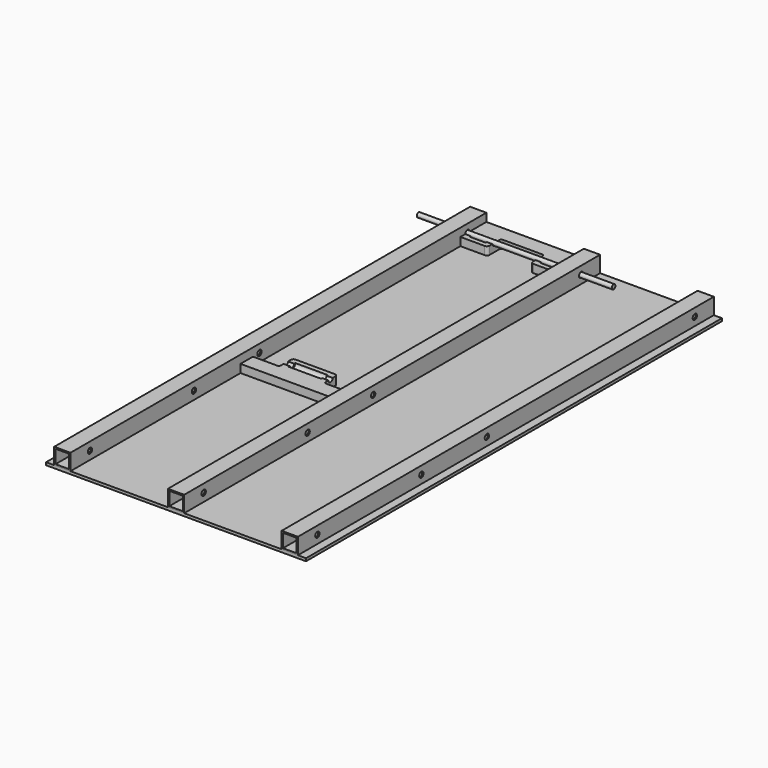
from build123d import *

# Parameters (mm, degrees)
F0_W      = 1219.2
F0_H      = 2438.4
F1_DEPTH  = 12.7
F2_W      = 76.2
F2_H      = 76.2
F2_W_2    = 63.5
F2_H_2    = 63.5
F3_DEPTH  = 1219.2
F5_DEPTH  = 76.2
F6_R      = 12.7
F7_DEPTH  = 609.6
F8_R      = 9.525
F8_2_R    = 9.525
F9_R      = 12.7
F9_2_R    = 12.7
F11_R     = 10.668
F12_DEPTH = 457.2
F14_W     = 1451.5540599823
F14_H     = 2822.6795196533
F15_DEPTH = 38.101
F17_R     = 19.05
F18_DEPTH = 38.1
F19_R     = 3.175
F20_R     = 19.05
F21_DEPTH = 76.2


# Not quite as in the source:
# - a pattern or mirror of a feature is missing from the dataset's text; its kind, count and spacing are read off the source's solid


with BuildPart() as f1:
    # F0 (on Top) → F1 (new body)
    with BuildSketch(Plane.XY):
        Rectangle(F0_W, F0_H)
    extrude(amount=F1_DEPTH)


with BuildPart() as f3:
    # F2 (on Front) → F3 (new body, symmetric)
    with BuildSketch(Plane.XZ):
        with Locations((0, 50.8)):
            Rectangle(F2_W, F2_H)
        with Locations((0, 50.8)):
            Rectangle(F2_W_2, F2_H_2, mode=Mode.SUBTRACT)
    extrude(amount=F3_DEPTH, both=True)


with BuildPart() as f3b:
    # F2 (on Front) → F3, piece 2 (new body, symmetric)
    with BuildSketch(Plane.XZ):
        with Locations((-533.4, 50.8)):
            Rectangle(F2_W, F2_H)
        with Locations((-533.4, 50.8)):
            Rectangle(F2_W_2, F2_H_2, mode=Mode.SUBTRACT)
    extrude(amount=F3_DEPTH, both=True)


with BuildPart() as f3c:
    # F2 (on Front) → F3, piece 3 (new body, symmetric)
    with BuildSketch(Plane.XZ):
        with Locations((533.4, 50.8)):
            Rectangle(F2_W, F2_H)
        with Locations((533.4, 50.8)):
            Rectangle(F2_W_2, F2_H_2, mode=Mode.SUBTRACT)
    extrude(amount=F3_DEPTH, both=True)


with BuildPart() as f5:
    # F4 (on face) → F5 (new body, through all)
    with BuildSketch(Plane.XY.offset(12.7)):
        Polygon((-495.3, 1219.2), (-495.3, 1066.8), (-368.3, 1066.8), (-368.3, 1146.175), (-165.1, 1146.175), (-165.1, 1066.8), (-38.1, 1066.8), (-38.1, 1219.2), align=None)
    extrude(amount=F5_DEPTH)


with BuildPart() as f5b:
    # F4 (on face) → F5, piece 2 (new body, through all)
    with BuildSketch(Plane.XY.offset(12.7)):
        Polygon((-495.3, -149.225), (-495.3, -222.25), (-38.1, -222.25), (-38.1, -149.225), (-161.925, -149.225), (-161.925, -69.85), (-371.475, -69.85), (-371.475, -149.225), align=None)
    extrude(amount=F5_DEPTH)


with BuildPart() as f7_tool:
    # F6 (on Right) → F7 (new body, symmetric)
    with BuildSketch(Plane.YZ):
        with Locations((1108.075, 50.8)):
            Circle(F6_R)
        with Locations((-111.125, 50.8)):
            Circle(F6_R)
        with Locations((-495.3, 50.8)):
            Circle(F6_R)
        with Locations((-1104.9, 50.8)):
            Circle(F6_R)
    extrude(amount=F7_DEPTH, both=True)


with BuildPart() as f3_1:
    add(f3.part)

    # F7: cut by f7_tool
    add(f7_tool.part, mode=Mode.SUBTRACT)


with BuildPart() as f3b_1:
    add(f3b.part)

    # F7: cut by f7_tool
    add(f7_tool.part, mode=Mode.SUBTRACT)


with BuildPart() as f3c_1:
    add(f3c.part)

    # F7: cut by f7_tool
    add(f7_tool.part, mode=Mode.SUBTRACT)


with BuildPart() as f5_1:
    add(f5.part)

    # F7: cut by f7_tool
    add(f7_tool.part, mode=Mode.SUBTRACT)

    # F8
    f8_edges = [f5_1.edges().sort_by_distance(p)[0] for p in [
        (-165.1, 1146.175, 50.8),
        (-368.3, 1146.175, 50.8),
    ]]
    fillet(f8_edges, radius=F8_R)

    # F9
    f9_edges = [f5_1.edges().sort_by_distance(p)[0] for p in [
        (-165.1, 1066.8, 50.8),
        (-368.3, 1066.8, 50.8),
    ]]
    fillet(f9_edges, radius=F9_R)


with BuildPart() as f5b_1:
    add(f5b.part)

    # F7: cut by f7_tool
    add(f7_tool.part, mode=Mode.SUBTRACT)

    # F8#2
    f8_2_edges = [f5b_1.edges().sort_by_distance(p)[0] for p in [
        (-371.475, -149.225, 50.8),
        (-161.925, -149.225, 50.8),
    ]]
    fillet(f8_2_edges, radius=F8_2_R)

    # F9#2
    f9_2_edges = [f5b_1.edges().sort_by_distance(p)[0] for p in [
        (-161.925, -69.85, 50.8),
        (-371.475, -69.85, 50.8),
    ]]
    fillet(f9_2_edges, radius=F9_2_R)


with BuildPart() as f12:
    # F11 (on offset) → F12 (new body, symmetric)
    with BuildSketch(Plane.YZ.offset(-266.7)):
        with Locations((1108.075, 50.8)):
            Circle(F11_R)
    extrude(amount=F12_DEPTH, both=True)


with BuildPart() as f15_tool:
    # F14 (on offset) → F15 (new body, through all)
    with BuildSketch(Plane.XY.offset(50.8)):
        Rectangle(F14_W, F14_H)
    extrude(amount=F15_DEPTH)


with BuildPart() as f5_2:
    add(f5_1.part)

    # F15: cut by f15_tool
    add(f15_tool.part, mode=Mode.SUBTRACT)

    # F17 (on offset) → F18 (cut, symmetric)
    with BuildSketch(Plane.YZ.offset(-101.6)):
        with Locations((1108.075, 50.8)):
            Circle(F17_R)
    f18 = extrude(amount=F18_DEPTH, both=True, mode=Mode.SUBTRACT)

    # F18_copies: F18 across plane
    add(f18.mirror(Plane(origin=(-266.7, 0, 0), x_dir=(0, 0, -1), z_dir=(-1, 0, 0))), mode=Mode.SUBTRACT)

    # F19
    f19_edges = [f5_2.edges().sort_by_distance(p)[0] for p in [
        (-139.7, 1108.075, 31.75),
        (-63.5, 1108.075, 31.75),
        (-393.7, 1108.075, 31.75),
        (-469.9, 1108.075, 31.75),
    ]]
    fillet(f19_edges, radius=F19_R)


with BuildPart() as f5b_2:
    add(f5b_1.part)

    # F15: cut by f15_tool
    add(f15_tool.part, mode=Mode.SUBTRACT)

    # F20 (on offset) → F21 (cut, symmetric)
    with BuildSketch(Plane.YZ.offset(-266.7)):
        with Locations((-111.125, 50.8)):
            Circle(F20_R)
    extrude(amount=F21_DEPTH, both=True, mode=Mode.SUBTRACT)


solid = Compound([f1.part, f3_1.part, f3b_1.part, f3c_1.part, f12.part, f5_2.part, f5b_2.part])
